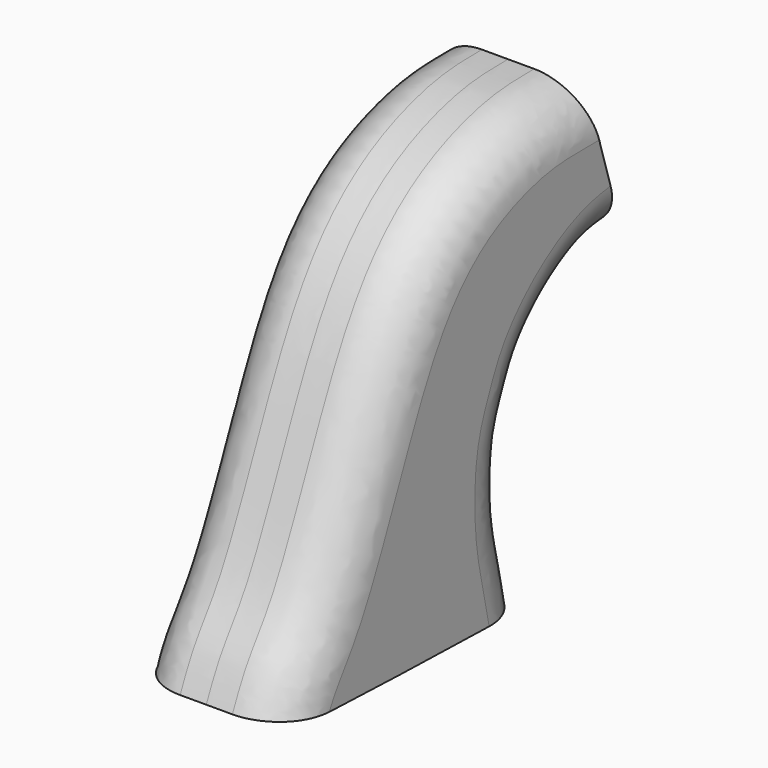
from build123d import *

# Parameters (mm, degrees)
F1_DEPTH = 7.62
F2_DEPTH = 7.62
F3_R     = 5.08


with BuildPart() as f1:
    # F0 (on Right) → F1 (new body)
    with BuildSketch(Plane.YZ):
        with BuildLine():
            Line((-6.3758171163, -10.4619786143), (-10.8449310064, 4.0714615025))
            add(Edge.make_bspline(
                [(-10.8449310064, 4.0714615025), (-12.6221476189, 4.0634001872), (-16.4526393634, 4.0460253769), (-23.6380003526, 1.7388194639), (-29.7987846192, -2.7378448885), (-35.4319131711, -10.9239362606), (-41.8175453088, -27.7803431947), (-45.7222383354, -32.2484724836), (-46.9524239971, -35.0151058711), (-47.5122109056, -36.2740419805)],
                knots=[0, 0, 0, 0, 0.1196163426, 0.2578129248, 0.3947257809, 0.5577277613, 0.773276306, 0.8968310559, 1, 1, 1, 1], degree=3))
            add(Edge.make_bspline(
                [(-47.5122109056, -36.2740419805), (-45.9109635043, -36.3972263768), (-41.0376251898, -36.7721336135), (-26.924120065, -37.1011760213), (-17.447931692, -37.3221039772)],
                knots=[0, 0, 0, 0, 0.3285730023, 1, 1, 1, 1], degree=3))
            add(Edge.make_bspline(
                [(-17.447931692, -37.3221039772), (-17.7505420436, -35.833321268), (-18.3539428771, -32.8647092467), (-19.4071863185, -28.7274264701), (-19.3765863034, -22.3807817014), (-17.9887341264, -19.2950416588), (-16.7856566039, -16.2235072113), (-13.488094812, -12.8738129326), (-9.6121048148, -10.7433586726), (-7.3935247559, -10.5504635272), (-6.3758171163, -10.4619786143)],
                knots=[0, 0, 0, 0, 0.1293800439, 0.2579820085, 0.4101867574, 0.5221864366, 0.6310245566, 0.7631794881, 0.8913656313, 1, 1, 1, 1], degree=3))
        make_face()
    extrude(amount=F1_DEPTH)

    # F0 (on Right) → F2 (join)
    with BuildSketch(Plane.YZ):
        with BuildLine():
            Line((-6.3758171163, -10.4619786143), (-10.8449310064, 4.0714615025))
            add(Edge.make_bspline(
                [(-10.8449310064, 4.0714615025), (-12.6221476189, 4.0634001872), (-16.4526393634, 4.0460253769), (-23.6380003526, 1.7388194639), (-29.7987846192, -2.7378448885), (-35.4319131711, -10.9239362606), (-41.8175453088, -27.7803431947), (-45.7222383354, -32.2484724836), (-46.9524239971, -35.0151058711), (-47.5122109056, -36.2740419805)],
                knots=[0, 0, 0, 0, 0.1196163426, 0.2578129248, 0.3947257809, 0.5577277613, 0.773276306, 0.8968310559, 1, 1, 1, 1], degree=3))
            add(Edge.make_bspline(
                [(-47.5122109056, -36.2740419805), (-45.9109635043, -36.3972263768), (-41.0376251898, -36.7721336135), (-26.924120065, -37.1011760213), (-17.447931692, -37.3221039772)],
                knots=[0, 0, 0, 0, 0.3285730023, 1, 1, 1, 1], degree=3))
            add(Edge.make_bspline(
                [(-17.447931692, -37.3221039772), (-17.7505420436, -35.833321268), (-18.3539428771, -32.8647092467), (-19.4071863185, -28.7274264701), (-19.3765863034, -22.3807817014), (-17.9887341264, -19.2950416588), (-16.7856566039, -16.2235072113), (-13.488094812, -12.8738129326), (-9.6121048148, -10.7433586726), (-7.3935247559, -10.5504635272), (-6.3758171163, -10.4619786143)],
                knots=[0, 0, 0, 0, 0.1293800439, 0.2579820085, 0.4101867574, 0.5221864366, 0.6310245566, 0.7631794881, 0.8913656313, 1, 1, 1, 1], degree=3))
        make_face()
    extrude(amount=-F2_DEPTH)

    # F3
    f3_edges = [f1.edges().sort_by_distance(p)[0] for p in [
        (-7.62, -34.401989, -10.194619),
        (-7.62, -18.563493, -20.649537),
        (7.62, -34.401989, -10.194619),
        (7.62, -18.563493, -20.649537),
    ]]
    fillet(f3_edges, radius=F3_R)


solid = f1.part
